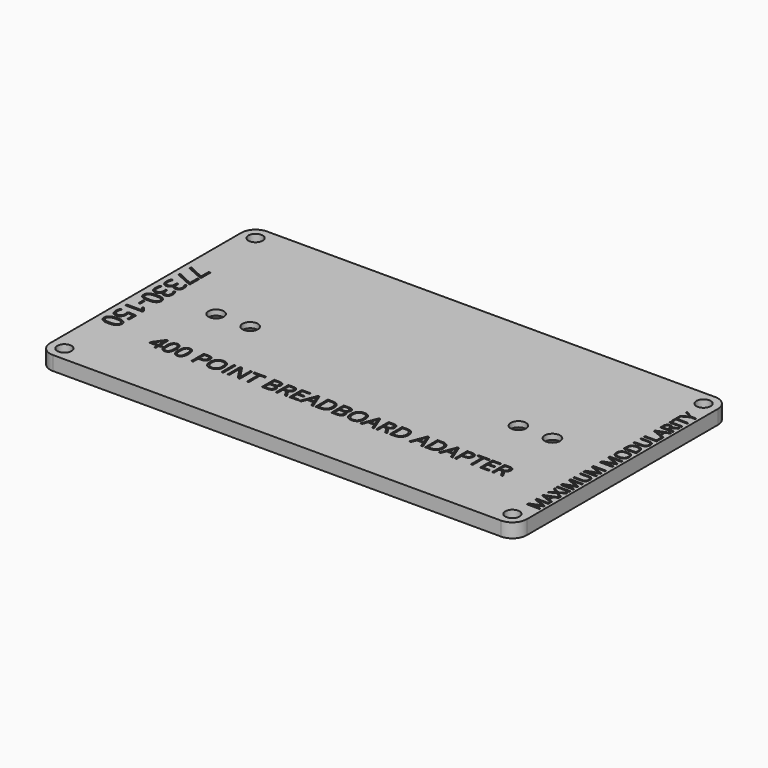
from build123d import *

# Parameters (mm, degrees)
F0_R           = 1.524
F1_DEPTH       = 2.9972
F2_TEXT_SIZE   = 5.172457681
F2_TEXT_SIZE_2 = 4.6394900823
F2_TEXT_SIZE_3 = 3.7383764187
F3_DEPTH       = 0.254
F4_D           = 3.2639
F4_CSINK_D     = 6.477
F4_CSINK_ANGLE = 82


# Not quite as in the source:
# - Text() gives the source's letters only with a copy of the font that has no kerning and outlines rounded to 1/6400 em; it was checked with that copy


with BuildPart() as f1:
    # F0 (on Top) → F1 (new body)
    with BuildSketch(Plane.XY):
        with BuildLine():
            ThreePointArc((0, 3.048), (0.8927385309, 0.8927385309), (3.048, 0))
            Line((3.048, 0), (98.298, 0))
            ThreePointArc((98.298, 0), (100.4532614691, 0.8927385309), (101.346, 3.048))
            Line((101.346, 3.048), (101.346, 53.848))
            ThreePointArc((101.346, 53.848), (100.4532614691, 56.0032614691), (98.298, 56.896))
            Line((98.298, 56.896), (3.048, 56.896))
            ThreePointArc((3.048, 56.896), (0.8927385309, 56.0032614691), (0, 53.848))
            Line((0, 53.848), (0, 3.048))
        make_face()
        with Locations((3.048, 3.048)):
            Circle(F0_R, mode=Mode.SUBTRACT)
        with Locations((98.298, 3.048)):
            Circle(F0_R, mode=Mode.SUBTRACT)
        with Locations((3.048, 53.848)):
            Circle(F0_R, mode=Mode.SUBTRACT)
        with Locations((98.298, 53.848)):
            Circle(F0_R, mode=Mode.SUBTRACT)
    extrude(amount=F1_DEPTH)

    # F2 (on face) → F3 (cut)
    with BuildSketch(Plane.XY.offset(2.9972)):
        with Locations(Location((1.27, 39.7002), (0, 0, -90))):
            Text('77330-150', F2_TEXT_SIZE, font='Open Sans', text_align=(TextAlign.LEFT, TextAlign.BOTTOM))
        with Locations((12.7, 12.7)):
            Text('400 POINT BREADBOARD ADAPTER', F2_TEXT_SIZE_2, font='Open Sans', text_align=(TextAlign.LEFT, TextAlign.BOTTOM))
        with Locations(Location((100.711, 6.858), (0, 0, 90))):
            Text('MAXIMUM MODULARITY', F2_TEXT_SIZE_3, font='Open Sans', text_align=(TextAlign.LEFT, TextAlign.BOTTOM))
    extrude(amount=-F3_DEPTH, mode=Mode.SUBTRACT)

    # F4 (through all)
    with Locations(Plane(origin=(0, 0, 0), x_dir=(1, 0, 0), z_dir=(0, 0, -1))):
        with Locations((14.986, -28.448), (86.487, -28.448), (22.225, -28.448), (79.248, -28.448)):
            CounterSinkHole(F4_D / 2, F4_CSINK_D / 2, counter_sink_angle=F4_CSINK_ANGLE)


solid = f1.part
